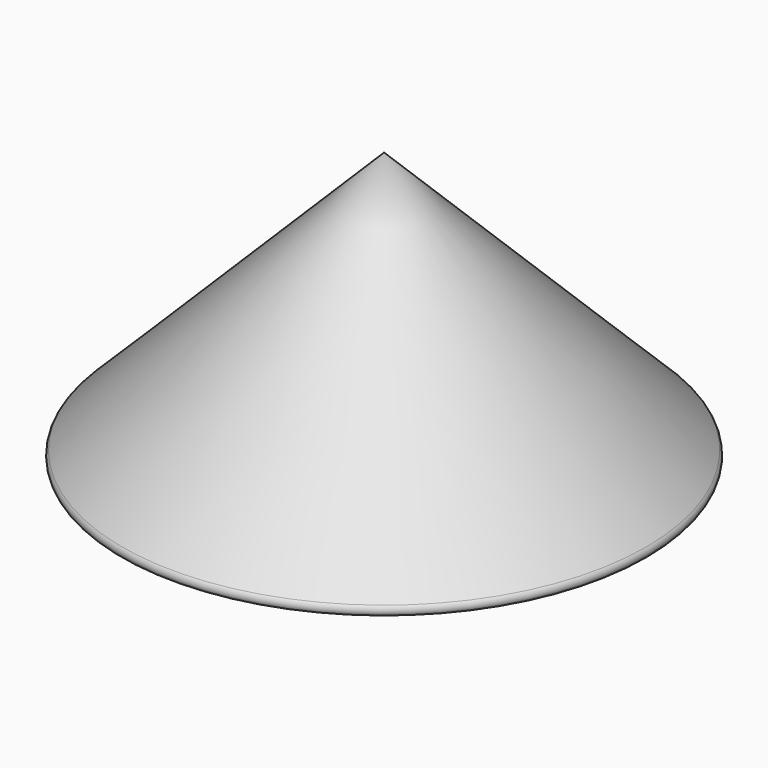
from build123d import *

# Parameters (mm, degrees)
F2_T = -5


# Not quite as in the source:
# - a fillet or chamfer that OpenCascade refuses, or shapes differently, is made with other operations: its cross-section is extruded or revolved along the edge and cut away or added
# - a feature of the source that left no trace in its solid (it failed there, or was rolled back) is left out


with BuildPart() as f1:
    # F0 (on Front) → F1 (revolve)
    with BuildSketch(Plane.XZ):
        Polygon((0, 210), (0, 0), (210, 0), align=None)
    revolve(axis=Axis((0, 0, 105), (0, 0, 1)))

    # F2
    f2_openings = [f1.faces().sort_by_distance(p)[0] for p in [
        (0, 0, 0),
    ]]
    offset(amount=F2_T, openings=f2_openings)

    # F3: fillet of radius 5 on 1 edges, made by hand

    # F3_s1 → F3_t2 (revolve, cut)
    with BuildSketch(Plane.XZ):
        with BuildLine():
            ThreePointArc((202.9289321881, 7.0710678119), (204.3933982822, 3.5355339059), (202.9289321881, 0))
            Line((202.9289321881, 0), (210, 0))
            Line((210, 0), (202.9289321881, 7.0710678119))
        make_face()
    revolve(axis=Axis((0, 0, 0), (0, 0, 1)), mode=Mode.SUBTRACT)


solid = f1.part
